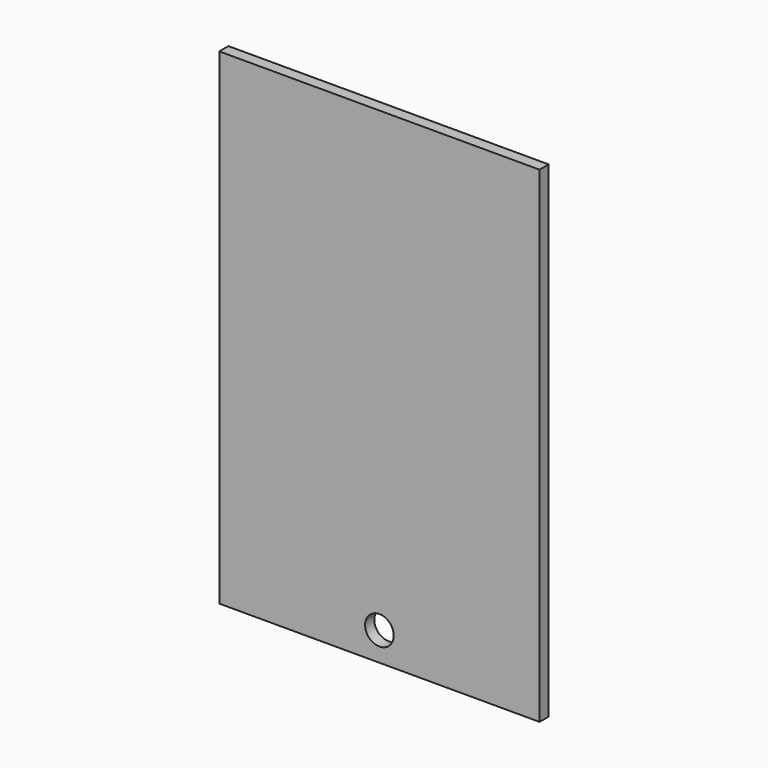
from build123d import *

# Parameters (mm, degrees)
F0_W     = 224
F0_H     = 340
F1_DEPTH = 8
F2_R     = 10
F3_DEPTH = 8


# Not quite as in the source:
# - a feature names something its author has since deleted; it is built from what else it names


with BuildPart() as f1:
    # F0 (on Front) → F1 (new body)
    with BuildSketch(Plane.XZ):
        Rectangle(F0_W, F0_H)
    extrude(amount=F1_DEPTH)

    # F2 (on face) → F3 (cut, through all)
    with BuildSketch(Plane.XZ.offset(8)):
        with Locations((0, -150)):
            Circle(F2_R)
    extrude(amount=-F3_DEPTH, mode=Mode.SUBTRACT)


solid = f1.part
